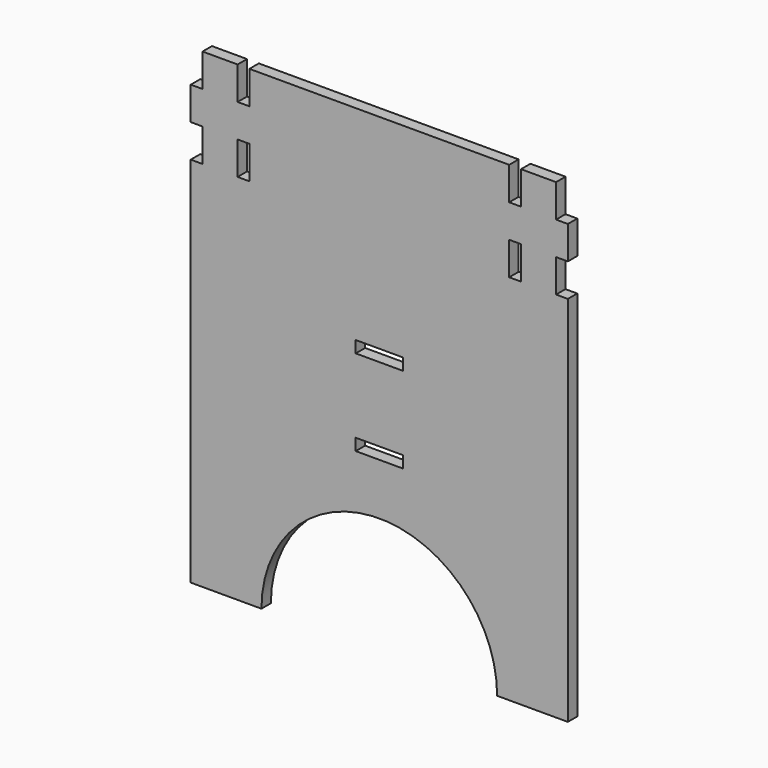
from build123d import *

# Parameters (mm, degrees)
F0_W     = 3.175
F0_H     = 8.89
F0_H_2   = 12.7
F0_H_3   = 49.53
F0_H_4   = 27.94
F0_W_2   = 8.89
F0_H_5   = 11.43
F0_W_3   = 12.7
F0_H_6   = 3.175
F1_DEPTH = 3.175


with BuildPart() as f1:
    # F0 (on Front) → F1 (new body)
    with BuildSketch(Plane.XZ):
        with BuildLine():
            Line((-38.175, 76.2), (-47.625, 76.2))
            Line((-47.625, 76.2), (-47.625, 67.31))
            Line((-47.625, 67.31), (-47.625, 58.42))
            Line((-47.625, 58.42), (-47.625, 49.53))
            Line((-47.625, 49.53), (-47.625, 40.64))
            Line((-47.625, 40.64), (-47.625, 27.94))
            Line((-47.625, 27.94), (-47.625, 0))
            Line((-47.625, 0), (-50.8, 0))
            Line((-50.8, 0), (-50.8, -50.8))
            Line((-50.8, -50.8), (-43.18, -50.8))
            Line((-43.18, -50.8), (-43.18, -41.91))
            Line((-43.18, -41.91), (-34.29, -41.91))
            Line((-34.29, -41.91), (-34.29, -50.8))
            Line((-34.29, -50.8), (-31.75, -50.8))
            ThreePointArc((-31.75, -50.8), (0, -19.05), (31.75, -50.8))
            Line((31.75, -50.8), (50.8, -50.8))
            Line((50.8, -50.8), (50.8, 0))
            Line((50.8, 0), (47.625, 0))
            Line((47.625, 0), (47.625, 12.7))
            Line((47.625, 12.7), (47.625, 25.4))
            Line((47.625, 25.4), (47.625, 38.1))
            Line((47.625, 38.1), (47.625, 49.53))
            Line((47.625, 49.53), (47.625, 58.42))
            Line((47.625, 58.42), (47.625, 67.31))
            Line((47.625, 67.31), (47.625, 76.2))
            Line((47.625, 76.2), (38.175, 76.2))
            Line((38.175, 76.2), (38.175, 67.31))
            Line((38.175, 67.31), (38.175, 58.42))
            Line((38.175, 58.42), (38.175, 49.53))
            Line((38.175, 49.53), (38.175, 40.64))
            Line((38.175, 40.64), (38.175, 27.94))
            Line((38.175, 27.94), (38.175, 0))
            Line((38.175, 0), (35, 0))
            Line((35, 0), (35, 27.94))
            Line((35, 27.94), (35, 40.64))
            Line((35, 40.64), (35, 49.53))
            Line((35, 49.53), (35, 58.42))
            Line((35, 58.42), (35, 67.31))
            Line((35, 67.31), (35, 76.2))
            Line((35, 76.2), (-35, 76.2))
            Line((-35, 76.2), (-35, 67.31))
            Line((-35, 67.31), (-35, 58.42))
            Line((-35, 58.42), (-35, 49.53))
            Line((-35, 49.53), (-35, 0))
            Line((-35, 0), (-38.175, 0))
            Line((-38.175, 0), (-38.175, 49.53))
            Line((-38.175, 49.53), (-38.175, 58.42))
            Line((-38.175, 58.42), (-38.175, 67.31))
            Line((-38.175, 67.31), (-38.175, 76.2))
        make_face()
        Polygon((19.05, -1.975), (31.75, -1.975), (31.75, -5.15), (19.05, -5.15), (6.35, -5.15), (-6.35, -5.15), (-19.05, -5.15), (-31.75, -5.15), (-31.75, -1.975), (-19.05, -1.975), (-6.35, -1.975), (6.35, -1.975), align=None, mode=Mode.SUBTRACT)
        Polygon((19.05, 21.2), (31.75, 21.2), (31.75, 18.025), (19.05, 18.025), (6.35, 18.025), (-6.35, 18.025), (-19.05, 18.025), (-31.75, 18.025), (-31.75, 21.2), (-19.05, 21.2), (-6.35, 21.2), (6.35, 21.2), align=None, mode=Mode.SUBTRACT)
        with Locations((-49.2125, 62.865)):
            Rectangle(F0_W, F0_H)
        with Locations((-36.5875, 62.865)):
            Rectangle(F0_W, F0_H)
        with Locations((-49.2125, 45.085)):
            Rectangle(F0_W, F0_H)
        with Locations((-49.2125, 34.29)):
            Rectangle(F0_W, F0_H_2)
        with Locations((36.5875, 62.865)):
            Rectangle(F0_W, F0_H)
        with Locations((-36.5875, 24.765)):
            Rectangle(F0_W, F0_H_3)
        with Locations((-49.2125, 13.97)):
            Rectangle(F0_W, F0_H_4)
        with Locations((49.2125, 62.865)):
            Rectangle(F0_W, F0_H)
        with Locations((36.5875, 45.085)):
            Rectangle(F0_W, F0_H)
        with Locations((36.5875, 34.29)):
            Rectangle(F0_W, F0_H_2)
        with Locations((-38.735, -46.355)):
            Rectangle(F0_W_2, F0_H)
        with Locations((49.2125, 43.815)):
            Rectangle(F0_W, F0_H_5)
        with Locations((36.5875, 13.97)):
            Rectangle(F0_W, F0_H_4)
        with Locations((49.2125, 31.75)):
            Rectangle(F0_W, F0_H_2)
        with Locations((49.2125, 19.05)):
            Rectangle(F0_W, F0_H_2)
        with Locations((49.2125, 6.35)):
            Rectangle(F0_W, F0_H_2)
        with Locations((25.4, 19.6125)):
            Rectangle(F0_W_3, F0_H_6)
        with Locations((12.7, 19.6125)):
            Rectangle(F0_W_3, F0_H_6)
        with Locations((-12.7, 19.6125)):
            Rectangle(F0_W_3, F0_H_6)
        with Locations((-25.4, 19.6125)):
            Rectangle(F0_W_3, F0_H_6)
        with Locations((25.4, -3.5625)):
            Rectangle(F0_W_3, F0_H_6)
        with Locations((12.7, -3.5625)):
            Rectangle(F0_W_3, F0_H_6)
        with Locations((-12.7, -3.5625)):
            Rectangle(F0_W_3, F0_H_6)
        with Locations((-25.4, -3.5625)):
            Rectangle(F0_W_3, F0_H_6)
    extrude(amount=F1_DEPTH)


solid = f1.part
